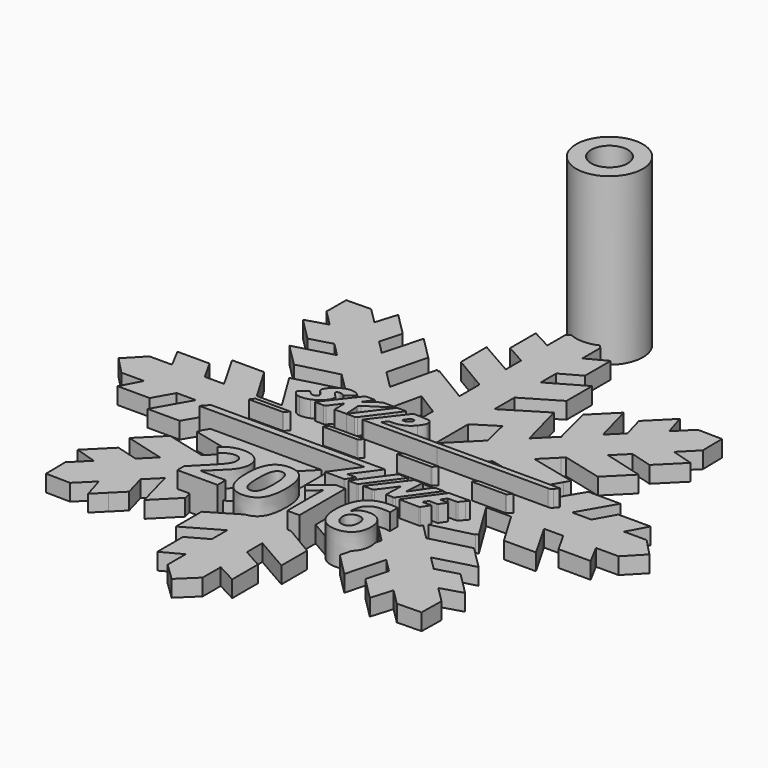
from build123d import *

# Parameters (mm, degrees)
F1_DEPTH     = 5.08
F3_DEPTH     = 2.54
F4_TEXT_SIZE = 12.3472222222
F5_DEPTH     = 5.08
F6_R         = 5.108655409
F6_R_2       = 2.8118150751
F7_DEPTH     = 25.4


# Not quite as in the source:
# - ends of sketch curves that miss each other by under 0.0002 mm in the source are joined
# - Text() gives the source's letters only with a copy of the font that has no kerning and outlines rounded to 1/6400 em; it was checked with that copy


with BuildPart() as f1:
    # F0 (on Top) → F1 (new body)
    with BuildSketch(Plane.XY):
        with BuildLine():
            add(Edge.make_bspline(
                [(10.7758714212, -9.2931907012), (10.7910997112, -9.3077512759), (10.8118855799, -9.3111949389)],
                knots=[4.110214, 4.110214, 4.110214, 4.709019, 4.709019, 4.709019], degree=2, weights=[1, 0.9555128919, 1]))
            Line((10.7758714212, -9.2931907012), (10.9943013235, -6.3281572082))
            ThreePointArc((10.9943013235, -6.3281572082), (10.4529610703, -6.3279623425), (9.9116490085, -6.3224308679))
            ThreePointArc((9.9116490085, -6.3224308679), (9.7363298723, -6.3543883378), (9.6055770182, -6.4754744939))
            Line((9.6055770182, -6.4754744939), (6.0316586945, -11.1746701971))
            ThreePointArc((6.0316586945, -11.1746701971), (5.9601349467, -11.2785407131), (5.8876130181, -11.3817167135))
            ThreePointArc((5.8876130181, -11.3817167135), (6.5649368046, -11.3778160466), (7.2422516166, -11.3817283176))
            ThreePointArc((7.2422516166, -11.3817283176), (7.4076659697, -11.3513321532), (7.5393230967, -11.2466852009))
            Line((7.5393230967, -11.2466852009), (9.5155478972, -8.5730061672))
            Line((9.5155478972, -8.5730061672), (9.407520325, -11.3871244224))
            ThreePointArc((9.407520325, -11.3871244224), (9.9477144109, -11.3886068187), (10.4877959466, -11.3997310312))
            ThreePointArc((10.4877959466, -11.3997310312), (10.6427379511, -11.3650321926), (10.7578725232, -11.2556954156))
            Line((10.7578725232, -11.2556954156), (14.1427289054, -6.5384868913))
            ThreePointArc((14.1427289054, -6.5384868913), (14.2020914745, -6.4535450248), (14.2597546815, -6.3674405524))
            ThreePointArc((14.2597546815, -6.3674405524), (13.6467919787, -6.359358131), (13.0337718925, -6.3592737316))
            ThreePointArc((13.0337718925, -6.3592737316), (12.8413417761, -6.4264815828), (12.6843548956, -6.5564899787))
            Line((12.6843548956, -6.5564899787), (10.8118855799, -9.3111949389))
        make_face()
    extrude(amount=F1_DEPTH)


with BuildPart() as f1b:
    # F0 (on Top) → F1, piece 2 (new body)
    with BuildSketch(Plane.XY):
        with BuildLine():
            ThreePointArc((15.7901540951, -7.600764776), (15.871674004, -7.5630631149), (15.9611922007, -7.5557553612))
            ThreePointArc((15.9611922007, -7.5557553612), (16.5256603447, -7.561264084), (17.0901532853, -7.5600078715))
            ThreePointArc((17.0901532853, -7.5600078715), (17.2062037369, -7.5512248061), (17.3115333632, -7.5017266998))
            ThreePointArc((17.3115333632, -7.5017266998), (17.6215719905, -7.1404609266), (17.9236891079, -6.772542757))
            ThreePointArc((17.9236891079, -6.772542757), (18.0911849699, -6.5707748368), (18.2567855411, -6.3674485561))
            ThreePointArc((18.2567855411, -6.3674485561), (18.1804059251, -6.3604511923), (18.1037399302, -6.3584478455))
            Line((18.1037399302, -6.3584478455), (15.2140023295, -6.3854478307))
            ThreePointArc((15.2140023295, -6.3854478307), (15.0590604251, -6.4201432773), (14.9439258531, -6.5294800542))
            Line((14.9439258531, -6.5294800542), (12.5043107274, -9.878339331))
            Line((12.5043107274, -9.878339331), (11.442039601, -11.3457138531))
            Line((11.442039601, -11.3457138531), (11.5860763639, -11.3817230438))
            Line((11.5860763639, -11.3817230438), (14.493818515, -11.3997276392))
            ThreePointArc((14.493818515, -11.3997276392), (14.5635843386, -11.3817190769), (14.6198477041, -11.3367091222))
            Line((14.6198477041, -11.3367091222), (15.3850459854, -10.1844174522))
            Line((15.3850459854, -10.1844174522), (13.9899419091, -10.1844174522))
            Line((13.9899419091, -10.1844174522), (14.0617082263, -10.0853921777))
            ThreePointArc((14.0617082263, -10.0853921777), (14.23230077, -9.8314556666), (14.3947960269, -9.5722628961))
            ThreePointArc((14.3947960269, -9.5722628961), (14.4984521828, -9.4655609687), (14.6468574919, -9.4552316147))
            Line((14.6468574919, -9.4552316147), (15.709614826, -9.4694009565))
            ThreePointArc((15.709614826, -9.4694009565), (15.8059195624, -9.4429985754), (15.8733417734, -9.3693369484))
            Line((15.8733417734, -9.3693369484), (16.5373400886, -8.3929602136))
            Line((16.5373400886, -8.3929602136), (15.2590138179, -8.3659533206))
            ThreePointArc((15.2590138179, -8.3659533206), (15.5221188384, -7.9816462236), (15.7901540951, -7.600764776))
        make_face()
    extrude(amount=F1_DEPTH)


with BuildPart() as f1c:
    # F0 (on Top) → F1, piece 3 (new body)
    with BuildSketch(Plane.XY):
        with BuildLine():
            Line((-10.5325690391, 5.4615759179), (-9.2812496614, 6.5238470443))
            ThreePointArc((-9.2812496614, 6.5238470443), (-9.4347707562, 6.6492938847), (-9.5873189586, 6.7759219257))
            ThreePointArc((-9.5873189586, 6.7759219257), (-10.1776898709, 7.0560035013), (-10.829644876, 7.0999942069))
            add(Edge.make_bspline(
                [(-13.4133042971, 5.488582811), (-12.7831434594, 6.3978148768), (-11.945929775, 6.9829642261), (-10.829644876, 7.0999942069)],
                knots=[0, 0, 0, 0, 1, 1, 1, 1], degree=3))
            ThreePointArc((-13.4133042971, 5.488582811), (-13.5122974671, 5.3025567147), (-13.5753455121, 5.10148398))
            ThreePointArc((-13.5753455121, 5.10148398), (-13.5819943862, 4.8010441602), (-13.4133024706, 4.552346178))
            ThreePointArc((-13.4133024706, 4.552346178), (-13.1272380052, 4.2403272243), (-12.8821740248, 3.8951728403))
            ThreePointArc((-12.8821740248, 3.8951728403), (-12.8452219795, 3.6784977417), (-12.972192263, 3.4990758993))
            ThreePointArc((-12.972192263, 3.4990758993), (-13.483605699, 3.2986595243), (-13.998452276, 3.4900742861))
            ThreePointArc((-13.998452276, 3.4900742861), (-14.2045136189, 3.6707692853), (-14.4035503772, 3.8591737084))
            Line((-14.4035503772, 3.8591737084), (-15.5018373592, 2.9319302695))
            ThreePointArc((-15.5018373592, 2.9319302695), (-15.6116796694, 2.7580339678), (-15.5468535589, 2.562831563))
            ThreePointArc((-15.5468535589, 2.562831563), (-15.0982093172, 2.131386393), (-14.5025827971, 1.9506716778))
            ThreePointArc((-14.5025827971, 1.9506716778), (-13.7346063631, 1.9950651493), (-12.9991995881, 2.22075097))
            ThreePointArc((-12.9991995881, 2.22075097), (-12.0419658498, 2.7397417289), (-11.2887601437, 3.5260805914))
            ThreePointArc((-11.2887601437, 3.5260805914), (-11.0941837405, 3.9466207812), (-11.0547116416, 4.4083062583))
            ThreePointArc((-11.0547116416, 4.4083062583), (-11.1061446162, 4.5471546675), (-11.189738089, 4.6693725593))
            ThreePointArc((-11.189738089, 4.6693725593), (-11.4120860811, 4.9017438852), (-11.6308541106, 5.1374888565))
            add(Edge.make_bspline(
                [(-11.3697827234, 5.7496494437), (-11.8379022029, 5.7046379553), (-11.918922882, 5.4975851087), (-11.6308541106, 5.1374888565)],
                knots=[0, 0, 0, 0, 1, 1, 1, 1], degree=3))
            ThreePointArc((-11.3697827234, 5.7496494437), (-11.159640755, 5.7463251988), (-10.9556719428, 5.6956492832))
            ThreePointArc((-10.9556719428, 5.6956492832), (-10.7398404169, 5.5863474448), (-10.5325690391, 5.4615759179))
        make_face()
    extrude(amount=F1_DEPTH)


with BuildPart() as f1d:
    # F0 (on Top) → F1, piece 4 (new body)
    with BuildSketch(Plane.XY):
        with BuildLine():
            ThreePointArc((-2.7005614911, 2.8689073654), (-2.5731537321, 3.0403845575), (-2.4574982279, 3.2199979446))
            add(Edge.make_bspline(
                [(-2.4574982279, 3.2199979446), (-2.2954666607, 3.5530888095), (-2.0524046233, 3.6431117863), (-1.6833104184, 3.6431117863)],
                knots=[0, 0, 0, 0, 1, 1, 1, 1], degree=3))
            add(Edge.make_bspline(
                [(-1.6833104184, 3.6431117863), (-0.5310163151, 3.6341094886), (0.4502341321, 4.0122059912), (1.1974248397, 4.9304403547)],
                knots=[0, 0, 0, 0, 1, 1, 1, 1], degree=3))
            add(Edge.make_bspline(
                [(1.1974248397, 4.9304403547), (1.4584914724, 5.2545230713), (1.7105558075, 5.5786057878), (1.7915764866, 6.0017137788)],
                knots=[0, 0, 0, 0, 1, 1, 1, 1], degree=3))
            add(Edge.make_bspline(
                [(1.7915764866, 6.0017137788), (1.8815994634, 6.4878378536), (1.6475397237, 6.8479297609), (1.1614156489, 6.8839389516)],
                knots=[0, 0, 0, 0, 1, 1, 1, 1], degree=3))
            ThreePointArc((1.1614156489, 6.8839389516), (0.1354491758, 6.9356869761), (-0.8911082928, 6.9739596368))
            ThreePointArc((-0.8911082928, 6.9739596368), (-1.0817861776, 6.9354416888), (-1.2241901704, 6.8029164084))
            Line((-1.2241901704, 6.8029164084), (-4.7981054161, 2.1397280735))
            ThreePointArc((-4.7981054161, 2.1397280735), (-4.8544834301, 2.0602835361), (-4.9061339224, 1.9776872622))
            Line((-4.9061339224, 1.9776872622), (-4.6450663555, 1.9776867153))
            Line((-4.6450663555, 1.9776867153), (6.5447896624, 1.9866890129))
            Line((6.5447896624, 1.9866890129), (6.5627942577, 1.9866890129))
            Line((6.5627942577, 1.9866890129), (23.532125387, 1.9866890129))
            ThreePointArc((23.532125387, 1.9866890129), (23.8729300003, 2.0430090536), (24.1442823062, 2.2567574268))
            ThreePointArc((24.1442823062, 2.2567574268), (24.3847706583, 2.5377063565), (24.6394155789, 2.8058905264))
            Line((24.6394155789, 2.8058905264), (24.6214034064, 2.8689141857))
            Line((24.6214034064, 2.8689141857), (-2.7005614911, 2.8689073654))
        make_face()
        with BuildLine():
            add(Edge.make_bspline(
                [(-1.1701794505, 4.8764265687), (-0.675053078, 4.6783760197), (0.0451307365, 5.0834794153), (0.1171491179, 5.5966103832)],
                knots=[0, 0, 0, 0, 1, 1, 1, 1], degree=3))
            Line((-1.1701794505, 4.8764265687), (-0.5940323989, 5.6686287646))
            add(Edge.make_bspline(
                [(0.0721376295, 5.7316448484), (-0.053894538, 5.8576770159), (-0.4950071244, 5.8126655275), (-0.5940323989, 5.6686287646)],
                knots=[0, 0, 0, 0, 1, 1, 1, 1], degree=3))
            ThreePointArc((0.0721376295, 5.7316448484), (0.1118644678, 5.6698679804), (0.1171491179, 5.5966103832))
        make_face(mode=Mode.SUBTRACT)
    extrude(amount=F1_DEPTH)


with BuildPart() as f1e:
    # F0 (on Top) → F1, piece 5 (new body)
    with BuildSketch(Plane.XY):
        with BuildLine():
            Line((-12.9091756269, -1.7492645248), (-18.2205312589, -1.7492645248))
            ThreePointArc((-18.2205312589, -1.7492645248), (-18.2844497675, -1.7577217602), (-18.3375739852, -1.794264441))
            Line((-18.3375739852, -1.794264441), (-18.7876760128, -2.3884276602))
            Line((-18.7876760128, -2.3884276602), (-13.6203571438, -2.3884276602))
            ThreePointArc((-13.6203571438, -2.3884276602), (-13.5455479941, -2.3815861375), (-13.4763153415, -2.3524266468))
            ThreePointArc((-13.4763153415, -2.3524266468), (-13.1913888623, -2.0521194957), (-12.9091756269, -1.7492645248))
        make_face()
    extrude(amount=F1_DEPTH)


with BuildPart() as f1f:
    # F0 (on Top) → F1, piece 6 (new body)
    with BuildSketch(Plane.XY):
        with BuildLine():
            Line((21.2185348829, -1.7402622271), (15.9251838463, -1.7402622271))
            ThreePointArc((15.9251838463, -1.7402622271), (15.8436778296, -1.7531403459), (15.7721487938, -1.7942807276))
            Line((15.7721487938, -1.7942807276), (15.3490367947, -2.3794253625))
            Line((15.3490367947, -2.3794253625), (20.5163556638, -2.3794253625))
            ThreePointArc((20.5163556638, -2.3794253625), (20.572211086, -2.3814699969), (20.6243896531, -2.3614308174))
            ThreePointArc((20.6243896531, -2.3614308174), (20.924614804, -2.0538600346), (21.2185348829, -1.7402622271))
        make_face()
    extrude(amount=F1_DEPTH)


with BuildPart() as f1g:
    # F0 (on Top) → F1, piece 7 (new body)
    with BuildSketch(Plane.XY):
        with BuildLine():
            ThreePointArc((-6.1034388113, 1.9596798311), (-5.920139748, 1.9911846096), (-5.779357055, 2.1127219743))
            Line((-5.779357055, 2.1127219743), (-3.7538388851, 4.8314150802))
            Line((-3.7538388851, 4.8314150802), (-2.1694344931, 6.955957333))
            ThreePointArc((-2.1694344931, 6.955957333), (-2.7726393352, 6.9536383345), (-3.3757421233, 6.9649682354))
            ThreePointArc((-3.3757421233, 6.9649682354), (-3.549031772, 6.9289384), (-3.6818136003, 6.8119159517))
            Line((-3.6818136003, 6.8119159517), (-7.1116959202, 2.2657602411))
            ThreePointArc((-7.1116959202, 2.2657602411), (-7.2201204521, 2.1175110274), (-7.3277447721, 1.9686798933))
            ThreePointArc((-7.3277447721, 1.9686798933), (-6.7155443901, 1.9710421087), (-6.1034388113, 1.9596798311))
        make_face()
    extrude(amount=F1_DEPTH)


with BuildPart() as f1h:
    # F0 (on Top) → F1, piece 8 (new body)
    with BuildSketch(Plane.XY):
        with BuildLine():
            ThreePointArc((-7.8048676931, 5.5786127659), (-7.8162355639, 5.5905356179), (-7.8228690155, 5.6056147494))
            ThreePointArc((-7.8228690155, 5.6056147494), (-7.3464374865, 6.2455816364), (-6.8812979904, 6.8938103137))
            ThreePointArc((-6.8812979904, 6.8938103137), (-6.9645541815, 6.9134319155), (-7.0486791413, 6.9289548028))
            ThreePointArc((-7.0486791413, 6.9289548028), (-7.6113234415, 6.9255835807), (-8.1739670317, 6.9289516823))
            ThreePointArc((-8.1739670317, 6.9289516823), (-8.3660074132, 6.8993676995), (-8.5160549503, 6.7759117971))
            Line((-8.5160549503, 6.7759117971), (-11.4418011049, 3.0129509486))
            ThreePointArc((-11.4418011049, 3.0129509486), (-11.8230745313, 2.5171943644), (-12.2110731292, 2.0266833822))
            ThreePointArc((-12.2110731292, 2.0266833822), (-12.0551714521, 2.0135808336), (-11.8995858136, 1.9972228507))
            ThreePointArc((-11.8995858136, 1.9972228507), (-11.3645486169, 1.9987376931), (-10.8296446022, 1.9866964132))
            ThreePointArc((-10.8296446022, 1.9866964132), (-10.663793388, 2.0076718249), (-10.5415698012, 2.1217226244))
            Line((-10.5415698012, 2.1217226244), (-9.3082565544, 3.7601416562))
            ThreePointArc((-9.3082565544, 3.7601416562), (-9.2649278532, 3.8025217799), (-9.2182354716, 3.8411648273))
            Line((-9.2182354716, 3.8411648273), (-9.1552174938, 3.8321600376))
            Line((-9.1552174938, 3.8321600376), (-9.1552174938, 1.9686844176))
            Line((-9.1552174938, 1.9686844176), (-7.3367533622, 1.9686844176))
            Line((-7.3367533622, 1.9686844176), (-7.4987947205, 4.2372634333))
            ThreePointArc((-7.4987947205, 4.2372634333), (-7.4586437444, 4.4910163793), (-7.2737408634, 4.6693812552))
            Line((-7.2737408634, 4.6693812552), (-4.0329101132, 6.7399021887))
            ThreePointArc((-4.0329101132, 6.7399021887), (-3.8924633433, 6.8554195038), (-3.7628445685, 6.9829673734))
            Line((-3.7628445685, 6.9829673734), (-5.7523489703, 6.9829642261))
            ThreePointArc((-5.7523489703, 6.9829642261), (-5.8427214761, 6.9584752354), (-5.923402269, 6.9109581166))
            Line((-5.923402269, 6.9109581166), (-6.9316499666, 6.1997643278))
            Line((-6.9316499666, 6.1997643278), (-7.8048676931, 5.5786127659))
        make_face()
    extrude(amount=F1_DEPTH)


with BuildPart() as f1i:
    # F0 (on Top) → F1, piece 9 (new body)
    with BuildSketch(Plane.XY):
        with BuildLine():
            Line((0.0271261411, -11.3637184484), (2.9618751852, -11.3637184484))
            ThreePointArc((2.9618751852, -11.3637184484), (3.0246589404, -11.3523116368), (3.0789014541, -11.3187030339))
            ThreePointArc((3.0789014541, -11.3187030339), (3.4691392597, -10.7446665082), (3.8531124905, -10.1664193108))
            ThreePointArc((3.8531124905, -10.1664193108), (3.1644709287, -10.1551729771), (2.4757511668, -10.1574148836))
            Line((2.4757511668, -10.1574148836), (5.2574610939, -6.376445533))
            Line((5.2574610939, -6.376445533), (-21.3920407321, -6.3584409376))
            ThreePointArc((-21.3920407321, -6.3584409376), (-21.8778535339, -6.8791240061), (-22.3505919982, -7.4117057724))
            Line((-22.3505919982, -7.4117057724), (2.9348682922, -7.4117097663))
            Line((2.9348682922, -7.4117097663), (0.0271261411, -11.3637184484))
        make_face()
    extrude(amount=F1_DEPTH)


with BuildPart() as f1j:
    # F0 (on Top) → F1, piece 10 (new body)
    with BuildSketch(Plane.XY):
        with BuildLine():
            Line((8.7323479989, -6.3584409376), (7.4630240259, -6.3584409376))
            ThreePointArc((7.4630240259, -6.3584409376), (7.3194269626, -6.3863246351), (7.210956034, -6.4844707945))
            Line((7.210956034, -6.4844707945), (3.7270704881, -11.2556908763))
            ThreePointArc((3.7270704881, -11.2556908763), (3.6882927093, -11.3263249636), (3.6550636239, -11.3997323262))
            Line((3.6550636239, -11.3997323262), (5.0053967589, -11.3997276392))
            ThreePointArc((5.0053967589, -11.3997276392), (5.0972963187, -11.368015903), (5.1674455247, -11.3007073229))
            ThreePointArc((5.1674455247, -11.3007073229), (5.5206961473, -10.8296925626), (5.86961036, -10.3554560247))
            Line((5.86961036, -10.3554560247), (8.7413502966, -6.4214570214))
            Line((8.7413502966, -6.4214570214), (8.7323479989, -6.3584409376))
        make_face()
    extrude(amount=F1_DEPTH)


with BuildPart() as f1k:
    # F0 (on Top) → F1, piece 11 (new body)
    with BuildSketch(Plane.XY):
        with BuildLine():
            Line((-1.6112920369, -1.7492645248), (-6.8236223944, -1.7492645248))
            ThreePointArc((-6.8236223944, -1.7492645248), (-6.9058746449, -1.7668497513), (-6.9766587791, -1.8122834771))
            Line((-6.9766587791, -1.8122834771), (-7.426776339, -2.3704230648))
            Line((-7.426776339, -2.3704230648), (-2.2324505769, -2.3704230648))
            ThreePointArc((-2.2324505769, -2.3704230648), (-2.1670503682, -2.3680440862), (-2.1064140552, -2.3434231115))
            ThreePointArc((-2.1064140552, -2.3434231115), (-1.8267290133, -2.064800596), (-1.5572755903, -1.7762738141))
            Line((-1.5572755903, -1.7762738141), (-1.6112920369, -1.7492645248))
        make_face()
    extrude(amount=F1_DEPTH)


with BuildPart() as f1l:
    # F0 (on Top) → F1, piece 12 (new body)
    with BuildSketch(Plane.XY):
        with BuildLine():
            Line((9.7316030416, -1.7582668225), (4.5192726841, -1.7582668225))
            ThreePointArc((4.5192726841, -1.7582668225), (4.4370204335, -1.7758520489), (4.3662362993, -1.8212857748))
            Line((4.3662362993, -1.8212857748), (3.9161187394, -2.3794253625))
            Line((3.9161187394, -2.3794253625), (9.1104445015, -2.3794253625))
            ThreePointArc((9.1104445015, -2.3794253625), (9.1758447103, -2.3770463838), (9.2364810233, -2.3524254092))
            ThreePointArc((9.2364810233, -2.3524254092), (9.5093040294, -2.0671586977), (9.7856165236, -1.7852734138))
            Line((9.7856165236, -1.7852734138), (9.7316030416, -1.7582668225))
        make_face()
    extrude(amount=F1_DEPTH)


with BuildPart() as f3:
    # F2 (on Top) → F3 (new body)
    with BuildSketch(Plane.XY):
        Polygon((38.0527542173, -2.6939323974), (40.6384947958, -0.0142280654), (40.6323866032, 0.0015361922), (38.0461705366, 2.6878242048), (34.5912743831, 2.6878242048), (36.2107500971, 5.7256807646), (31.2836697964, 5.7256807646), (29.5828856263, 2.6878242048), (26.629885395, 2.6878242048), (29.7241055764, 8.0756889996), (24.8066813407, 8.0756889996), (21.6057689566, 2.6878242048), (17.7678123168, 2.6878242048), (20.9311245691, 8.170164817), (21.4208406821, 9.0175210938), (14.4729361793, 10.6807051321), (16.7259082766, 12.9367496137), (17.1780242578, 13.3888655949), (23.250152929, 11.8414811841), (26.7238491484, 15.3156894676), (20.730468613, 16.9473815667), (22.8138012054, 19.0276417748), (26.1782814778, 18.0832859363), (29.6580858898, 21.5605300281), (26.360137368, 22.5643584484), (28.7985498039, 25.0058066926), (28.7324935412, 28.740106938), (24.9981932958, 28.8061632006), (22.5567450517, 26.3616425722), (21.5493687589, 29.6565552857), (18.0690522829, 26.179786682), (19.0169925697, 22.8218900902), (16.930112105, 20.7350462015), (15.3045281985, 26.7350469935), (11.8308319791, 23.2613141981), (13.3807401341, 17.1891855269), (10.6664714786, 14.4714055751), (8.7772477377, 21.5290380889), (3.9385350619, 18.5633459843), (2.679698744, 17.7947378435), (2.679698744, 21.619966034), (8.0741472194, 24.8208784181), (8.0741472194, 29.7352668455), (2.679698744, 26.6440824724), (2.679698744, 29.5940468954), (5.7241389844, 31.2979034498), (5.7241389844, 36.2153276855), (2.679698744, 34.5988877799), (2.679698744, 38.0542959974), (-0.0030413963, 40.64), (-2.6862936006, 38.0542959974), (-2.6862936006, 34.5988877799), (-5.7332941613, 36.2153276855), (-5.7332941613, 34.8091998009), (-5.7332941613, 31.2979034498), (-2.6862936006, 29.5940468954), (-2.6862936006, 26.6440824724), (-8.0777062678, 29.7352668455), (-8.0777062678, 24.8208784181), (-4.2864937607, 22.5709421291), (-2.6832577923, 21.619966034), (-2.6832577923, 17.7789735859), (-8.6172023217, 21.3690180729), (-8.6578382618, 21.2212144421), (-9.0124060412, 21.4315264632), (-10.6756266556, 14.4840974484), (-10.6756266556, 14.4805495761), (-13.3872984147, 17.1922579112), (-11.8369147717, 23.2643865824), (-15.3141588634, 26.7380828018), (-16.9361948976, 20.7380820098), (-19.0230753623, 22.8249624745), (-18.0817553322, 26.1828224903), (-19.239459, 27.3435985424), (-21.5554515515, 29.659591094), (-22.0355115996, 28.100026874), (-22.5628278443, 26.3616425722), (-25.0138955774, 28.8061632006), (-28.7761764656, 28.7339987454), (-28.7919041472, 25.909526591), (-28.8076684048, 25.0027343083), (-26.3662201606, 22.5612860641), (-29.6610962981, 21.5569821557), (-26.1843276944, 18.080250128), (-22.8264676786, 19.0246059665), (-20.739587214, 16.9443457584), (-26.7365521977, 15.3121415952), (-25.870395855, 14.4459852526), (-23.259783594, 11.8353729915), (-17.1841070504, 13.3822453382), (-15.0129188973, 11.2171653777), (-14.4729107793, 10.6710490671), (-21.5336156774, 8.7757171336), (-18.5272510567, 3.889748261), (-17.7932072393, 2.6878242048), (-20.3443834944, 2.6878242048), (-21.6153996215, 2.6878242048), (-24.2417395642, 7.1186047119), (-24.8127275573, 8.0792368719), (-29.730188369, 8.0792368719), (-28.8640320264, 6.5694525929), (-26.6425518683, 2.6908965891), (-29.5858960346, 2.6908965891), (-31.2933004613, 5.7287165729), (-36.2071768247, 5.7287165729), (-34.5973205997, 2.6908965891), (-38.0527653933, 2.6908965891), (-40.6384693958, 0.0045720005), (-38.0527653933, -2.6878242048), (-34.5973205997, -2.6878242048), (-36.2071768247, -5.7220963162), (-35.5076607548, -5.7220963162), (-31.2933004613, -5.7220963162), (-29.5858960346, -2.6878242048), (-26.6425518683, -2.6878242048), (-29.730188369, -8.0726166153), (-24.8127275573, -8.0726166153), (-21.6153996215, -2.6878242048), (-17.7774429817, -2.6878242048), (-21.3705232771, -8.6065165407), (-21.2232317103, -8.65988093), (-21.4269234747, -9.0109008371), (-14.4825668443, -10.6771572597), (-17.1841070504, -13.3857932106), (-23.259783594, -11.8384453758), (-26.7334798133, -15.3090692109), (-20.7365514057, -16.9377255018), (-22.8234318703, -19.0215335822), (-26.1812918861, -18.0771777437), (-29.6580604898, -21.5569821557), (-26.3631477763, -22.5582502558), (-28.8045960205, -25.0027343083), (-28.7385763339, -28.7370345537), (-25.02000377, -28.8061266246), (-25.0108597691, -28.8061266246), (-22.55975546, -26.3616425722), (-21.5524157432, -29.6565187097), (-19.8170672497, -27.9150985995), (-18.0786829479, -26.1767142977), (-19.020002978, -22.8188542819), (-16.9331590893, -20.7350462015), (-15.6306510231, -25.5518864272), (-15.3106109911, -26.7350104175), (-11.8338423874, -23.2455865166), (-13.3837505424, -17.179529462), (-10.669518463, -14.4617495102), (-9.0124060412, -21.1963061836), (-8.8869503487, -21.1241783044), (-8.7741499534, -21.5193820239), (-2.6862936006, -17.7916654592), (-2.679673344, -17.7850817785), (-2.679673344, -21.6138578414), (-8.0710860111, -24.8178426098), (-8.0710860111, -29.7322310372), (-2.679673344, -26.6380108558), (-2.679673344, -29.5910110871), (-5.7271859687, -31.2948310655), (-5.7271859687, -36.2153276855), (-2.679673344, -34.5993632679), (-2.679673344, -38.0512236131), (0.0030667963, -40.64), (2.6863190006, -38.0512236131), (2.6863190006, -34.5993632679), (5.730247177, -36.2153276855), (5.730247177, -31.2948310655), (2.6863190006, -29.5910110871), (2.6863190006, -28.6085430529), (2.6863190006, -26.6380108558), (7.8922913292, -29.6219909622), (8.0807674761, -29.7352668455), (8.0807674761, -24.8208784181), (2.6863190006, -21.6169302257), (2.6863190006, -20.7665381407), (2.6863190006, -17.7820459702), (7.0576635018, -20.3022057742), (9.0190516979, -21.4350743355), (10.3464314466, -15.8836416524), (10.6822357362, -14.4840974484), (13.3873238147, -17.1891855269), (11.8369035957, -23.2547305175), (15.3106363911, -26.7446664825), (16.9362202976, -20.7411178181), (18.329656309, -22.1315180212), (19.0231007623, -22.8249624745), (18.0756725396, -26.1828224903), (19.8140568414, -27.9212067921), (21.5554769515, -29.6631389663), (22.5628166683, -26.3677507648), (25.0042649124, -28.8122348172), (28.7386017339, -28.740106938), (28.8046214205, -25.0093545649), (26.3662455606, -22.5643584484), (29.6646695705, -21.5635658364), (28.619729722, -20.5155901796), (26.1843530944, -18.0832859363), (22.820384886, -19.0276417748), (20.7365768057, -16.9443457584), (26.730469405, -15.3156894676), (23.2562611216, -11.8450290565), (18.2763284956, -13.1063891186), (17.1841324504, -13.3888290189), (14.469900371, -10.6740848754), (21.2008725961, -9.0139366454), (21.1317805252, -8.8854085685), (21.5305686931, -8.7787529419), (17.7866123827, -2.6939323974), (21.6154250215, -2.6939323974), (24.4048573645, -7.3888648029), (24.8127529573, -8.0792368719), (29.730213769, -8.0792368719), (27.3014573981, -3.8455644486), (26.6359935876, -2.6939323974), (29.5889938189, -2.6939323974), (31.2933258613, -5.7287165729), (33.750501787, -5.7287165729), (36.2168582897, -5.7287165729), (35.0743702394, -3.5885082949), (34.5973459997, -2.6939323974), align=None)
        Polygon((-6.8661261466, -12.0705932711), (-7.1328017893, -10.9158888356), (-2.6954376015, -6.4815604562), (-2.6954376015, -12.7640011484), (-6.1914817591, -14.9671933047), align=None, mode=Mode.SUBTRACT)
        Polygon((-14.9626268923, -6.2118124292), (-12.7660184166, -2.6908600131), (-6.5054501745, -2.6908600131), (-10.9423022982, -7.1282607768), align=None, mode=Mode.SUBTRACT)
        Polygon((6.2072714167, -14.9545014315), (2.6736271274, -12.7518213392), (2.6736271274, -6.4815604562), (7.120135316, -10.9286172849), align=None, mode=Mode.SUBTRACT)
        Polygon((14.9626522923, -6.1772846817), (10.9083120148, -7.1186047119), (7.9552752075, -4.1625320963), (6.480055252, -2.6908600131), (12.7563877516, -2.6908600131), (14.0650040105, -4.7559046036), align=None, mode=Mode.SUBTRACT)
        Polygon((-14.8371346237, 5.9481725948), (-14.9814269581, 6.1772846817), (-10.9331582973, 7.1155689036), (-6.5023777902, 2.6847883965), (-12.7721266092, 2.6847883965), align=None, mode=Mode.SUBTRACT)
        Polygon((-3.1536617754, 13.0276775588), (-2.6954376015, 12.7579295318), (-2.6954376015, 6.4881807128), (-7.1424578542, 10.9286172849), (-6.2290818909, 14.9514656231), align=None, mode=Mode.SUBTRACT)
        Polygon((14.520192376, 6.3123964392), (14.9438522264, 6.2179206218), (12.7406600701, 2.6878242048), (6.480055252, 2.6878242048), (10.9143836314, 7.1252249685), align=None, mode=Mode.SUBTRACT)
        Polygon((2.6736271274, 12.7675855968), (6.1666354767, 14.970265689), (7.1079555068, 10.9189612199), (2.6736271274, 6.4881807128), align=None, mode=Mode.SUBTRACT)
    extrude(amount=F3_DEPTH)

    # F4 (on Top) → F5 (join)
    with BuildSketch(Plane.XY):
        with Locations((-14.5212217114, -22.0254785446)):
            Text('2016', F4_TEXT_SIZE, font='Open Sans', font_style=FontStyle.BOLD, text_align=(TextAlign.LEFT, TextAlign.BOTTOM))
    extrude(amount=F5_DEPTH)

    # F6 (on Top) → F7 (join)
    with BuildSketch(Plane.XY):
        with Locations((0, 43.1475639343)):
            Circle(F6_R)
        with Locations((0, 43.1475639343)):
            Circle(F6_R_2, mode=Mode.SUBTRACT)
    extrude(amount=F7_DEPTH)


solid = Compound([f1.part, f1b.part, f1c.part, f1d.part, f1e.part, f1f.part, f1g.part, f1h.part, f1i.part, f1j.part, f1k.part, f1l.part, f3.part])
